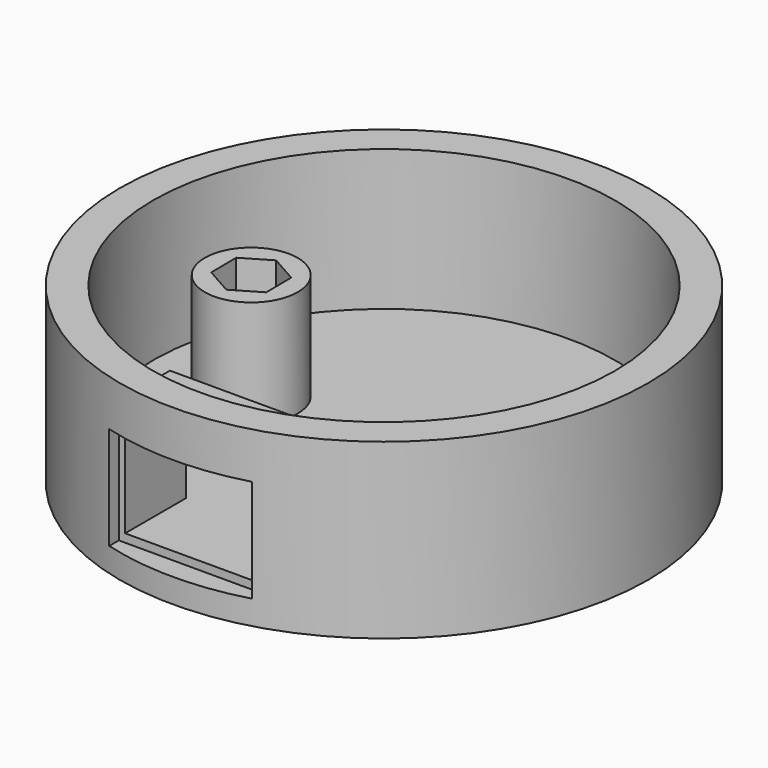
from build123d import *

# Parameters (mm, degrees)
F0_R     = 39.78873575
F0_R_2   = 34.78873575
F1_DEPTH = 26.1
F0_R_3   = 7
F0_R_4   = 3.5
F2_DEPTH = 4.9
F0_R_5   = 2.5
F3_DEPTH = 2
F4_DEPTH = 21
F6_START = 25
F5_W     = 19.6
F5_H     = 13
F6_DEPTH = 20
F7_START = 36.5
F5_W_2   = 21.5
F5_H_2   = 15.5
F7_DEPTH = 8.5
F8_START = 25
F8_DEPTH = 11.5
F9_START = 25
F9_DEPTH = 11.5


# Not quite as in the source:
# - a feature names something its author has since deleted; it is built from what else it names


with BuildPart() as f1:
    # F0 (on Top) → F1 (new body)
    with BuildSketch(Plane.XY):
        Circle(F0_R)
        Circle(F0_R_2, mode=Mode.SUBTRACT)
    extrude(amount=F1_DEPTH)

    # F0 (on Top) → F2 (join)
    with BuildSketch(Plane.XY):
        Circle(F0_R_2)
        with Locations((-20, 0)):
            Circle(F0_R_3, mode=Mode.SUBTRACT)
        Circle(F0_R_4, mode=Mode.SUBTRACT)
        Polygon((20, 4.1030999273), (20, 8), (25, 8), (25, 5), (25, -5), (25, -8), (20, -8), (20, -4.1030999273), align=None, mode=Mode.SUBTRACT)
    extrude(amount=F2_DEPTH)

    # F0 (on Top) → F3 (join)
    with BuildSketch(Plane.XY):
        Circle(F0_R_4)
        Circle(F0_R_5, mode=Mode.SUBTRACT)
    extrude(amount=F3_DEPTH)



with BuildPart() as f2:
    # F0 (on Top) → F2, piece 2 (new body)
    with BuildSketch(Plane.XY):
        Polygon((-24.1344178899, 2.3386082852), (-24.0925031294, -2.4112067799), (-19.9580852395, -4.7498150651), (-15.8655821101, -2.3386082852), (-15.9074968706, 2.4112067799), (-20.0419147605, 4.7498150651), align=None)
    extrude(amount=F2_DEPTH)


with BuildPart() as f1_1:
    add(f1.part)

    add(f2.part)  # F4 merges F2
    # F0 (on Top) → F4 (join)
    with BuildSketch(Plane.XY):
        with Locations((-20, 0)):
            Circle(F0_R_3)
        Polygon((-19.9580852395, -4.7498150651), (-24.0925031294, -2.4112067799), (-24.1344178899, 2.3386082852), (-20.0419147605, 4.7498150651), (-15.9074968706, 2.4112067799), (-15.8655821101, -2.3386082852), align=None, mode=Mode.SUBTRACT)
    extrude(amount=F4_DEPTH)

    # F5 (on Front) → F6 (cut)
    with BuildSketch(Plane.XZ.offset(F6_START)):
        with Locations((0, 11.4)):
            Rectangle(F5_W, F5_H)
    extrude(amount=F6_DEPTH, mode=Mode.SUBTRACT)

    # F5 (on Front) → F7 (cut)
    with BuildSketch(Plane.XZ.offset(F7_START)):
        with Locations((0, 11.4)):
            Rectangle(F5_W_2, F5_H_2)
        with Locations((0, 11.4)):
            Rectangle(F5_W, F5_H, mode=Mode.SUBTRACT)
    extrude(amount=F7_DEPTH, mode=Mode.SUBTRACT)

    # F5 (on Front) → F8 (join)
    with BuildSketch(Plane.XZ.offset(F8_START)):
        with Locations((0, 11.4)):
            Rectangle(F5_W_2, F5_H_2)
        with Locations((0, 11.4)):
            Rectangle(F5_W, F5_H, mode=Mode.SUBTRACT)
    extrude(amount=F8_DEPTH)

    # F5 (on Front) → F9 (join)
    with BuildSketch(Plane.XZ.offset(F9_START)):
        Polygon((-10.75, 3.65), (-10.75, 19.15), (10.75, 19.15), (10.75, 3.65), (12.25, 3.65), (12.25, 21), (-12.25, 21), (-12.25, 3.65), align=None)
    extrude(amount=F9_DEPTH)


solid = f1_1.part
